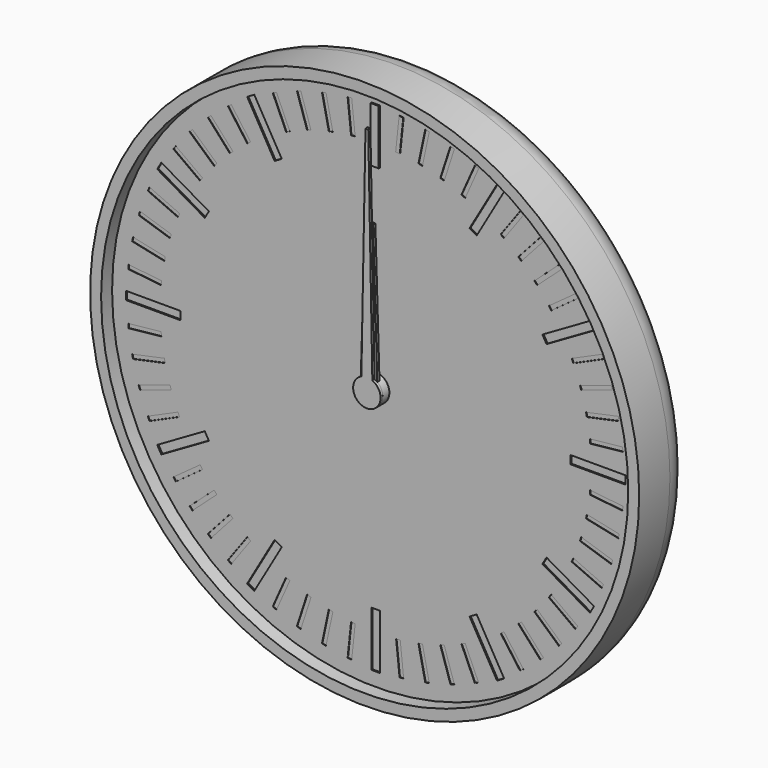
from build123d import *

# Parameters (mm, degrees)
F0_R      = 100
F1_DEPTH  = 24
F2_R      = 10
F3_T      = -4
F4_R      = 5
F4_R_2    = 3
F5_DEPTH  = 2
F6_DEPTH  = 19
F7_DEPTH  = 8
F9_DEPTH  = 4
F11_DEPTH = 4
F12_R     = 5
F12_R_2   = 3
F13_DEPTH = 2
F14_R     = 3
F15_DEPTH = 4
F17_DEPTH = 4
F18_R     = 3
F19_DEPTH = 2
F20_R     = 98
F20_R_2   = 5
F21_DEPTH = 1
F23_R     = 5
F23_R_2   = 3
F24_DEPTH = 2
F25_W     = 3
F25_H     = 20
F25_W_2   = 20
F25_H_2   = 3
F26_DEPTH = 0.5
F27_W     = 1.5
F27_H     = 12
F27_W_2   = 12
F27_H_2   = 1.5
F28_DEPTH = 0.2
F29_DEPTH = 1
F30_DEPTH = 0.4
F31_R     = 5
F31_R_2   = 3
F32_DEPTH = 5
F33_R     = 3
F34_DEPTH = 1
F36_DEPTH = 1


with BuildPart() as f1:
    # F0 (on Front) → F1 (new body)
    with BuildSketch(Plane.XZ):
        Circle(F0_R)
    extrude(amount=F1_DEPTH)

    # F2
    f2_edges = [f1.edges().sort_by_distance(p)[0] for p in [
        (-100, 0, 0),
    ]]
    fillet(f2_edges, radius=F2_R)

    # F3
    f3_openings = [f1.faces().sort_by_distance(p)[0] for p in [
        (0, -24, 0),
    ]]
    offset(amount=F3_T, openings=f3_openings)

    # F4 (on face) → F5 (join)
    with BuildSketch(Plane.XZ.offset(4)):
        Circle(F4_R)
        Circle(F4_R_2, mode=Mode.SUBTRACT)
        with Locations((40, 0)):
            Circle(F4_R)
        with Locations((40, 0)):
            Circle(F4_R_2, mode=Mode.SUBTRACT)
    extrude(amount=F5_DEPTH)


with BuildPart() as f6:
    # F6 (new): a face of the model
    f6_faces = [f1.part.faces().sort_by_distance(p)[0] for p in [
        (0, -4, 0),
    ]]
    extrude(f6_faces, amount=F6_DEPTH)

    # F8 (on face) → F9 (join)
    with BuildSketch(Plane.XZ.offset(6)):
        with BuildLine():
            ThreePointArc((9.2729637667, -1.3794085621), (9.3494561423, -0.6915886375), (9.375, 0))
            ThreePointArc((9.375, 0), (9.3494561423, 0.6915886375), (9.2729637667, 1.3794085621))
            ThreePointArc((9.2729637667, 1.3794085621), (8.9161548403, 2.8970343223), (8.3127812852, 4.3345463782))
            ThreePointArc((8.3127812852, 4.3345463782), (7.5845343223, 5.5104867402), (6.6911892658, 6.566476316))
            ThreePointArc((6.6911892658, 6.566476316), (5.5104867402, 7.5845343223), (4.1773988938, 8.3928519278))
            ThreePointArc((4.1773988938, 8.3928519278), (2.8970343223, 8.9161548403), (1.5536078905, 9.2453733036))
            ThreePointArc((1.5536078905, 9.2453733036), (0, 9.375), (-1.5536078905, 9.2453733036))
            ThreePointArc((-1.5536078905, 9.2453733036), (-2.8970343223, 8.9161548403), (-4.1773988938, 8.3928519278))
            ThreePointArc((-4.1773988938, 8.3928519278), (-5.5104867402, 7.5845343223), (-6.6911892658, 6.566476316))
            ThreePointArc((-6.6911892658, 6.566476316), (-7.5845343223, 5.5104867402), (-8.3127812852, 4.3345463782))
            ThreePointArc((-8.3127812852, 4.3345463782), (-8.9161548403, 2.8970343223), (-9.2729637667, 1.3794085621))
            ThreePointArc((-9.2729637667, 1.3794085621), (-9.375, 0), (-9.2729637667, -1.3794085621))
            ThreePointArc((-9.2729637667, -1.3794085621), (-8.9161548403, -2.8970343223), (-8.3127812852, -4.3345463782))
            ThreePointArc((-8.3127812852, -4.3345463782), (-7.5845343223, -5.5104867402), (-6.6911892658, -6.566476316))
            ThreePointArc((-6.6911892658, -6.566476316), (-5.5104867402, -7.5845343223), (-4.1773988938, -8.3928519278))
            ThreePointArc((-4.1773988938, -8.3928519278), (-2.8970343223, -8.9161548403), (-1.5536078905, -9.2453733036))
            ThreePointArc((-1.5536078905, -9.2453733036), (0, -9.375), (1.5536078905, -9.2453733036))
            ThreePointArc((1.5536078905, -9.2453733036), (2.8970343223, -8.9161548403), (4.1773988938, -8.3928519278))
            ThreePointArc((4.1773988938, -8.3928519278), (5.5104867402, -7.5845343223), (6.6911892658, -6.566476316))
            ThreePointArc((6.6911892658, -6.566476316), (7.5845343223, -5.5104867402), (8.3127812852, -4.3345463782))
            ThreePointArc((8.3127812852, -4.3345463782), (8.9161548403, -2.8970343223), (9.2729637667, -1.3794085621))
        make_face()
        with BuildLine():
            ThreePointArc((8.3127812852, 4.3345463782), (8.9161548403, 2.8970343223), (9.2729637667, 1.3794085621))
            Line((9.2729637667, 1.3794085621), (11.1823199426, 2.3946312492))
            Line((11.1823199426, 2.3946312492), (10.8182678729, 3.515068311))
            Line((10.8182678729, 3.515068311), (10.4542158031, 4.6355053728))
            Line((10.4542158031, 4.6355053728), (8.3127812852, 4.3345463782))
        make_face()
        with BuildLine():
            Line((11.1823199426, -2.3946312492), (9.2729637667, -1.3794085621))
            ThreePointArc((9.2729637667, -1.3794085621), (8.9161548403, -2.8970343223), (8.3127812852, -4.3345463782))
            Line((8.3127812852, -4.3345463782), (10.4542158031, -4.6355053728))
            Line((10.4542158031, -4.6355053728), (10.8182678729, -3.515068311))
            Line((10.8182678729, -3.515068311), (11.1823199426, -2.3946312492))
        make_face()
        with BuildLine():
            ThreePointArc((4.1773988938, 8.3928519278), (5.5104867402, 7.5845343223), (6.6911892658, 6.566476316))
            Line((6.6911892658, 6.566476316), (7.6391579371, 8.5101001246))
            Line((7.6391579371, 8.5101001246), (6.6860572448, 9.202568311))
            Line((6.6860572448, 9.202568311), (5.7329565525, 9.8950364974))
            Line((5.7329565525, 9.8950364974), (4.1773988938, 8.3928519278))
        make_face()
        with BuildLine():
            Line((7.6391579371, -8.5101001246), (6.6911892658, -6.566476316))
            ThreePointArc((6.6911892658, -6.566476316), (5.5104867402, -7.5845343223), (4.1773988938, -8.3928519278))
            Line((4.1773988938, -8.3928519278), (5.7329565525, -9.8950364974))
            Line((5.7329565525, -9.8950364974), (6.6860572448, -9.202568311))
            Line((6.6860572448, -9.202568311), (7.6391579371, -8.5101001246))
        make_face()
        with BuildLine():
            ThreePointArc((-1.5536078905, 9.2453733036), (0, 9.375), (1.5536078905, 9.2453733036))
            Line((1.5536078905, 9.2453733036), (1.1780972451, 11.375))
            Line((1.1780972451, 11.375), (0, 11.375))
            Line((0, 11.375), (-1.1780972451, 11.375))
            Line((-1.1780972451, 11.375), (-1.5536078905, 9.2453733036))
        make_face()
        with BuildLine():
            Line((1.1780972451, -11.375), (1.5536078905, -9.2453733036))
            ThreePointArc((1.5536078905, -9.2453733036), (0, -9.375), (-1.5536078905, -9.2453733036))
            Line((-1.5536078905, -9.2453733036), (-1.1780972451, -11.375))
            Line((-1.1780972451, -11.375), (0, -11.375))
            Line((0, -11.375), (1.1780972451, -11.375))
        make_face()
        with BuildLine():
            ThreePointArc((-6.6911892658, 6.566476316), (-5.5104867402, 7.5845343223), (-4.1773988938, 8.3928519278))
            Line((-4.1773988938, 8.3928519278), (-5.7329565525, 9.8950364974))
            Line((-5.7329565525, 9.8950364974), (-6.6860572448, 9.202568311))
            Line((-6.6860572448, 9.202568311), (-7.6391579371, 8.5101001246))
            Line((-7.6391579371, 8.5101001246), (-6.6911892658, 6.566476316))
        make_face()
        with BuildLine():
            Line((-5.7329565525, -9.8950364974), (-4.1773988938, -8.3928519278))
            ThreePointArc((-4.1773988938, -8.3928519278), (-5.5104867402, -7.5845343223), (-6.6911892658, -6.566476316))
            Line((-6.6911892658, -6.566476316), (-7.6391579371, -8.5101001246))
            Line((-7.6391579371, -8.5101001246), (-6.6860572448, -9.202568311))
            Line((-6.6860572448, -9.202568311), (-5.7329565525, -9.8950364974))
        make_face()
        with BuildLine():
            ThreePointArc((-9.2729637667, 1.3794085621), (-8.9161548403, 2.8970343223), (-8.3127812852, 4.3345463782))
            Line((-8.3127812852, 4.3345463782), (-10.4542158031, 4.6355053728))
            Line((-10.4542158031, 4.6355053728), (-10.8182678729, 3.515068311))
            Line((-10.8182678729, 3.515068311), (-11.1823199426, 2.3946312492))
            Line((-11.1823199426, 2.3946312492), (-9.2729637667, 1.3794085621))
        make_face()
        with BuildLine():
            Line((-10.4542158031, -4.6355053728), (-8.3127812852, -4.3345463782))
            ThreePointArc((-8.3127812852, -4.3345463782), (-8.9161548403, -2.8970343223), (-9.2729637667, -1.3794085621))
            Line((-9.2729637667, -1.3794085621), (-11.1823199426, -2.3946312492))
            Line((-11.1823199426, -2.3946312492), (-10.8182678729, -3.515068311))
            Line((-10.8182678729, -3.515068311), (-10.4542158031, -4.6355053728))
        make_face()
    extrude(amount=F9_DEPTH)

    # F35 (on face) → F36 (join)
    with BuildSketch(Plane.XZ.offset(23)):
        with BuildLine():
            ThreePointArc((-2, 4.582575695), (-2.7386127875, -4.1833001327), (5, 0))
            ThreePointArc((5, 0), (4.1833001327, 2.7386127875), (2, 4.582575695))
            ThreePointArc((2, 4.582575695), (0, 5), (-2, 4.582575695))
        make_face()
        with BuildLine():
            ThreePointArc((-2, 4.582575695), (0, 5), (2, 4.582575695))
            Line((2, 4.582575695), (0.5, 84.582575695))
            Line((0.5, 84.582575695), (0, 84.582575695))
            Line((0, 84.582575695), (-0.5, 84.582575695))
            Line((-0.5, 84.582575695), (-2, 4.582575695))
        make_face()
    extrude(amount=-F36_DEPTH)


with BuildPart() as f7:
    # F7 (new): a face of the model
    f7_faces = [f1.part.faces().sort_by_distance(p)[0] for p in [
        (40, -4, 0),
    ]]
    extrude(f7_faces, amount=F7_DEPTH)

    # F10 (on face) → F11 (join)
    with BuildSketch(Plane.XZ.offset(6)):
        with BuildLine():
            ThreePointArc((68.0829066802, -1.5381733945), (68.1144747006, -0.7693746225), (68.125, 0))
            ThreePointArc((68.125, 0), (68.1144747006, 0.7693746225), (68.0829066802, 1.5381733945))
            ThreePointArc((68.0829066802, 1.5381733945), (67.9709283072, 2.9398630294), (67.7890320221, 4.3342039956))
            ThreePointArc((67.7890320221, 4.3342039956), (67.5104012706, 5.8475163042), (67.1494235596, 7.3433252263))
            ThreePointArc((67.1494235596, 7.3433252263), (66.7484645208, 8.6911029668), (66.280643318, 10.0171558733))
            ThreePointArc((66.280643318, 10.0171558733), (65.6934659962, 11.4394680865), (65.0293803521, 12.8275385085))
            ThreePointArc((65.0293803521, 12.8275385085), (64.3569644814, 14.0625), (63.6236643925, 15.2623099717))
            ThreePointArc((63.6236643925, 15.2623099717), (62.7536029668, 16.5314602207), (61.815433119, 17.7511268046))
            ThreePointArc((61.815433119, 17.7511268046), (60.9009482166, 18.8192983038), (59.934217974, 19.8404278876))
            ThreePointArc((59.934217974, 19.8404278876), (58.8192983038, 20.9009482166), (57.6480467764, 21.8989056799))
            ThreePointArc((57.6480467764, 21.8989056799), (56.5314602207, 22.7536029668), (55.3735505752, 23.5514238999))
            ThreePointArc((55.3735505752, 23.5514238999), (54.0625, 24.3569644814), (52.709356105, 25.0895972944))
            ThreePointArc((52.709356105, 25.0895972944), (51.4394680865, 25.6934659962), (50.1409852457, 26.2331096755))
            ThreePointArc((50.1409852457, 26.2331096755), (48.6911029668, 26.7484645208), (47.2152055856, 27.1837531139))
            ThreePointArc((47.2152055856, 27.1837531139), (45.8475163042, 27.5104012706), (44.4652101991, 27.7682826779))
            ThreePointArc((44.4652101991, 27.7682826779), (42.9398630294, 27.9709283072), (41.4057159597, 28.0898484802))
            ThreePointArc((41.4057159597, 28.0898484802), (40, 28.125), (38.5942840403, 28.0898484802))
            ThreePointArc((38.5942840403, 28.0898484802), (37.0601369706, 27.9709283072), (35.5347898009, 27.7682826779))
            ThreePointArc((35.5347898009, 27.7682826779), (34.1524836958, 27.5104012706), (32.7847944144, 27.1837531139))
            ThreePointArc((32.7847944144, 27.1837531139), (31.3088970332, 26.7484645208), (29.8590147543, 26.2331096755))
            ThreePointArc((29.8590147543, 26.2331096755), (28.5605319135, 25.6934659962), (27.290643895, 25.0895972944))
            ThreePointArc((27.290643895, 25.0895972944), (25.9375, 24.3569644814), (24.6264494248, 23.5514238999))
            ThreePointArc((24.6264494248, 23.5514238999), (23.4685397793, 22.7536029668), (22.3519532236, 21.8989056799))
            ThreePointArc((22.3519532236, 21.8989056799), (21.1807016962, 20.9009482166), (20.065782026, 19.8404278876))
            ThreePointArc((20.065782026, 19.8404278876), (19.0990517834, 18.8192983038), (18.184566881, 17.7511268046))
            ThreePointArc((18.184566881, 17.7511268046), (17.2463970332, 16.5314602207), (16.3763356075, 15.2623099717))
            ThreePointArc((16.3763356075, 15.2623099717), (15.6430355186, 14.0625), (14.9706196479, 12.8275385085))
            ThreePointArc((14.9706196479, 12.8275385085), (14.3065340038, 11.4394680865), (13.719356682, 10.0171558733))
            ThreePointArc((13.719356682, 10.0171558733), (13.2515354792, 8.6911029668), (12.8505764404, 7.3433252263))
            ThreePointArc((12.8505764404, 7.3433252263), (12.4895987294, 5.8475163042), (12.2109679779, 4.3342039956))
            ThreePointArc((12.2109679779, 4.3342039956), (12.0290716928, 2.9398630294), (11.9170933198, 1.5381733945))
            ThreePointArc((11.9170933198, 1.5381733945), (11.875, 0), (11.9170933198, -1.5381733945))
            ThreePointArc((11.9170933198, -1.5381733945), (12.0290716928, -2.9398630294), (12.2109679779, -4.3342039956))
            ThreePointArc((12.2109679779, -4.3342039956), (12.4895987294, -5.8475163042), (12.8505764404, -7.3433252263))
            ThreePointArc((12.8505764404, -7.3433252263), (13.2515354792, -8.6911029668), (13.719356682, -10.0171558733))
            ThreePointArc((13.719356682, -10.0171558733), (14.3065340038, -11.4394680865), (14.9706196479, -12.8275385085))
            ThreePointArc((14.9706196479, -12.8275385085), (15.6430355186, -14.0625), (16.3763356075, -15.2623099717))
            ThreePointArc((16.3763356075, -15.2623099717), (17.2463970332, -16.5314602207), (18.184566881, -17.7511268046))
            ThreePointArc((18.184566881, -17.7511268046), (19.0990517834, -18.8192983038), (20.065782026, -19.8404278876))
            ThreePointArc((20.065782026, -19.8404278876), (21.1807016962, -20.9009482166), (22.3519532236, -21.8989056799))
            ThreePointArc((22.3519532236, -21.8989056799), (23.4685397793, -22.7536029668), (24.6264494248, -23.5514238999))
            ThreePointArc((24.6264494248, -23.5514238999), (25.9375, -24.3569644814), (27.290643895, -25.0895972944))
            ThreePointArc((27.290643895, -25.0895972944), (28.5605319135, -25.6934659962), (29.8590147543, -26.2331096755))
            ThreePointArc((29.8590147543, -26.2331096755), (31.3088970332, -26.7484645208), (32.7847944144, -27.1837531139))
            ThreePointArc((32.7847944144, -27.1837531139), (34.1524836958, -27.5104012706), (35.5347898009, -27.7682826779))
            ThreePointArc((35.5347898009, -27.7682826779), (37.0601369706, -27.9709283072), (38.5942840403, -28.0898484802))
            ThreePointArc((38.5942840403, -28.0898484802), (40, -28.125), (41.4057159597, -28.0898484802))
            ThreePointArc((41.4057159597, -28.0898484802), (42.9398630294, -27.9709283072), (44.4652101991, -27.7682826779))
            ThreePointArc((44.4652101991, -27.7682826779), (45.8475163042, -27.5104012706), (47.2152055856, -27.1837531139))
            ThreePointArc((47.2152055856, -27.1837531139), (48.6911029668, -26.7484645208), (50.1409852457, -26.2331096755))
            ThreePointArc((50.1409852457, -26.2331096755), (51.4394680865, -25.6934659962), (52.709356105, -25.0895972944))
            ThreePointArc((52.709356105, -25.0895972944), (54.0625, -24.3569644814), (55.3735505752, -23.5514238999))
            ThreePointArc((55.3735505752, -23.5514238999), (56.5314602207, -22.7536029668), (57.6480467764, -21.8989056799))
            ThreePointArc((57.6480467764, -21.8989056799), (58.8192983038, -20.9009482166), (59.934217974, -19.8404278876))
            ThreePointArc((59.934217974, -19.8404278876), (60.9009482166, -18.8192983038), (61.815433119, -17.7511268046))
            ThreePointArc((61.815433119, -17.7511268046), (62.7536029668, -16.5314602207), (63.6236643925, -15.2623099717))
            ThreePointArc((63.6236643925, -15.2623099717), (64.3569644814, -14.0625), (65.0293803521, -12.8275385085))
            ThreePointArc((65.0293803521, -12.8275385085), (65.6934659962, -11.4394680865), (66.280643318, -10.0171558733))
            ThreePointArc((66.280643318, -10.0171558733), (66.7484645208, -8.6911029668), (67.1494235596, -7.3433252263))
            ThreePointArc((67.1494235596, -7.3433252263), (67.5104012706, -5.8475163042), (67.7890320221, -4.3342039956))
            ThreePointArc((67.7890320221, -4.3342039956), (67.9709283072, -2.9398630294), (68.0829066802, -1.5381733945))
        make_face()
        with BuildLine():
            ThreePointArc((68.0829066802, 1.5381733945), (68.1144747006, 0.7693746225), (68.125, 0))
            ThreePointArc((68.125, 0), (68.1144747006, -0.7693746225), (68.0829066802, -1.5381733945))
            Line((68.0829066802, -1.5381733945), (70.125, -1.1780972451))
            Line((70.125, -1.1780972451), (70.125, 0))
            Line((70.125, 0), (70.125, 1.1780972451))
            Line((70.125, 1.1780972451), (68.0829066802, 1.5381733945))
        make_face()
        with BuildLine():
            ThreePointArc((67.1494235596, 7.3433252263), (67.5104012706, 5.8475163042), (67.7890320221, 4.3342039956))
            Line((67.7890320221, 4.3342039956), (69.7116366623, 5.1109866922))
            Line((69.7116366623, 5.1109866922), (69.4666964721, 6.2633396859))
            Line((69.4666964721, 6.2633396859), (69.2217562819, 7.4156926796))
            Line((69.2217562819, 7.4156926796), (67.1494235596, 7.3433252263))
        make_face()
        with BuildLine():
            Line((69.7116366623, -5.1109866922), (67.7890320221, -4.3342039956))
            ThreePointArc((67.7890320221, -4.3342039956), (67.5104012706, -5.8475163042), (67.1494235596, -7.3433252263))
            Line((67.1494235596, -7.3433252263), (69.2217562819, -7.4156926796))
            Line((69.2217562819, -7.4156926796), (69.4666964721, -6.2633396859))
            Line((69.4666964721, -6.2633396859), (69.7116366623, -5.1109866922))
        make_face()
        with BuildLine():
            ThreePointArc((65.0293803521, 12.8275385085), (65.6934659962, 11.4394680865), (66.280643318, 10.0171558733))
            Line((66.280643318, 10.0171558733), (67.9997322302, 11.1766959857))
            Line((67.9997322302, 11.1766959857), (67.5205569115, 12.2529413727))
            Line((67.5205569115, 12.2529413727), (67.0413815928, 13.3291867596))
            Line((67.0413815928, 13.3291867596), (65.0293803521, 12.8275385085))
        make_face()
        with BuildLine():
            Line((67.9997322302, -11.1766959857), (66.280643318, -10.0171558733))
            ThreePointArc((66.280643318, -10.0171558733), (65.6934659962, -11.4394680865), (65.0293803521, -12.8275385085))
            Line((65.0293803521, -12.8275385085), (67.0413815928, -13.3291867596))
            Line((67.0413815928, -13.3291867596), (67.5205569115, -12.2529413727))
            Line((67.5205569115, -12.2529413727), (67.9997322302, -11.1766959857))
        make_face()
        with BuildLine():
            ThreePointArc((61.815433119, 17.7511268046), (62.7536029668, 16.5314602207), (63.6236643925, 15.2623099717))
            Line((63.6236643925, 15.2623099717), (65.064105142, 16.753930033))
            Line((65.064105142, 16.753930033), (64.3716369555, 17.7070307253))
            Line((64.3716369555, 17.7070307253), (63.6791687691, 18.6601314176))
            Line((63.6791687691, 18.6601314176), (61.815433119, 17.7511268046))
        make_face()
        with BuildLine():
            Line((65.064105142, -16.753930033), (63.6236643925, -15.2623099717))
            ThreePointArc((63.6236643925, -15.2623099717), (62.7536029668, -16.5314602207), (61.815433119, -17.7511268046))
            Line((61.815433119, -17.7511268046), (63.6791687691, -18.6601314176))
            Line((63.6791687691, -18.6601314176), (64.3716369555, -17.7070307253))
            Line((64.3716369555, -17.7070307253), (65.064105142, -16.753930033))
        make_face()
        with BuildLine():
            ThreePointArc((57.6480467764, 21.8989056799), (58.8192983038, 20.9009482166), (59.934217974, 19.8404278876))
            Line((59.934217974, 19.8404278876), (61.0330563882, 21.5989369435))
            Line((61.0330563882, 21.5989369435), (60.1575595166, 22.3872378675))
            Line((60.1575595166, 22.3872378675), (59.282062645, 23.1755387915))
            Line((59.282062645, 23.1755387915), (57.6480467764, 21.8989056799))
        make_face()
        with BuildLine():
            Line((61.0330563882, -21.5989369435), (59.934217974, -19.8404278876))
            ThreePointArc((59.934217974, -19.8404278876), (58.8192983038, -20.9009482166), (57.6480467764, -21.8989056799))
            Line((57.6480467764, -21.8989056799), (59.282062645, -23.1755387915))
            Line((59.282062645, -23.1755387915), (60.1575595166, -22.3872378675))
            Line((60.1575595166, -22.3872378675), (61.0330563882, -21.5989369435))
        make_face()
        with BuildLine():
            ThreePointArc((52.709356105, 25.0895972944), (54.0625, 24.3569644814), (55.3735505752, 23.5514238999))
            Line((55.3735505752, 23.5514238999), (56.0827621424, 25.4999666665))
            Line((56.0827621424, 25.4999666665), (55.0625, 26.089015289))
            Line((55.0625, 26.089015289), (54.0422378576, 26.6780639116))
            Line((54.0422378576, 26.6780639116), (52.709356105, 25.0895972944))
        make_face()
        with BuildLine():
            Line((56.0827621424, -25.4999666665), (55.3735505752, -23.5514238999))
            ThreePointArc((55.3735505752, -23.5514238999), (54.0625, -24.3569644814), (52.709356105, -25.0895972944))
            Line((52.709356105, -25.0895972944), (54.0422378576, -26.6780639116))
            Line((54.0422378576, -26.6780639116), (55.0625, -26.089015289))
            Line((55.0625, -26.089015289), (56.0827621424, -25.4999666665))
        make_face()
        with BuildLine():
            ThreePointArc((47.2152055856, 27.1837531139), (48.6911029668, 26.7484645208), (50.1409852457, 26.2331096755))
            Line((50.1409852457, 26.2331096755), (50.4295740173, 28.2865254836))
            Line((50.4295740173, 28.2865254836), (49.3091369555, 28.6505775534))
            Line((49.3091369555, 28.6505775534), (48.1886998938, 29.0146296232))
            Line((48.1886998938, 29.0146296232), (47.2152055856, 27.1837531139))
        make_face()
        with BuildLine():
            Line((50.4295740173, -28.2865254836), (50.1409852457, -26.2331096755))
            ThreePointArc((50.1409852457, -26.2331096755), (48.6911029668, -26.7484645208), (47.2152055856, -27.1837531139))
            Line((47.2152055856, -27.1837531139), (48.1886998938, -29.0146296232))
            Line((48.1886998938, -29.0146296232), (49.3091369555, -28.6505775534))
            Line((49.3091369555, -28.6505775534), (50.4295740173, -28.2865254836))
        make_face()
        with BuildLine():
            ThreePointArc((41.4057159597, 28.0898484802), (42.9398630294, 27.9709283072), (44.4652101991, 27.7682826779))
            Line((44.4652101991, 27.7682826779), (44.3205634611, 29.8368274034))
            Line((44.3205634611, 29.8368274034), (43.1489199559, 29.959972098))
            Line((43.1489199559, 29.959972098), (41.9772764508, 30.0831167926))
            Line((41.9772764508, 30.0831167926), (41.4057159597, 28.0898484802))
        make_face()
        with BuildLine():
            Line((44.3205634611, -29.8368274034), (44.4652101991, -27.7682826779))
            ThreePointArc((44.4652101991, -27.7682826779), (42.9398630294, -27.9709283072), (41.4057159597, -28.0898484802))
            Line((41.4057159597, -28.0898484802), (41.9772764508, -30.0831167926))
            Line((41.9772764508, -30.0831167926), (43.1489199559, -29.959972098))
            Line((43.1489199559, -29.959972098), (44.3205634611, -29.8368274034))
        make_face()
        with BuildLine():
            ThreePointArc((35.5347898009, 27.7682826779), (37.0601369706, 27.9709283072), (38.5942840403, 28.0898484802))
            Line((38.5942840403, 28.0898484802), (38.0227235492, 30.0831167926))
            Line((38.0227235492, 30.0831167926), (36.8510800441, 29.959972098))
            Line((36.8510800441, 29.959972098), (35.6794365389, 29.8368274034))
            Line((35.6794365389, 29.8368274034), (35.5347898009, 27.7682826779))
        make_face()
        with BuildLine():
            Line((38.0227235492, -30.0831167926), (38.5942840403, -28.0898484802))
            ThreePointArc((38.5942840403, -28.0898484802), (37.0601369706, -27.9709283072), (35.5347898009, -27.7682826779))
            Line((35.5347898009, -27.7682826779), (35.6794365389, -29.8368274034))
            Line((35.6794365389, -29.8368274034), (36.8510800441, -29.959972098))
            Line((36.8510800441, -29.959972098), (38.0227235492, -30.0831167926))
        make_face()
        with BuildLine():
            ThreePointArc((29.8590147543, 26.2331096755), (31.3088970332, 26.7484645208), (32.7847944144, 27.1837531139))
            Line((32.7847944144, 27.1837531139), (31.8113001062, 29.0146296232))
            Line((31.8113001062, 29.0146296232), (30.6908630445, 28.6505775534))
            Line((30.6908630445, 28.6505775534), (29.5704259827, 28.2865254836))
            Line((29.5704259827, 28.2865254836), (29.8590147543, 26.2331096755))
        make_face()
        with BuildLine():
            Line((31.8113001062, -29.0146296232), (32.7847944144, -27.1837531139))
            ThreePointArc((32.7847944144, -27.1837531139), (31.3088970332, -26.7484645208), (29.8590147543, -26.2331096755))
            Line((29.8590147543, -26.2331096755), (29.5704259827, -28.2865254836))
            Line((29.5704259827, -28.2865254836), (30.6908630445, -28.6505775534))
            Line((30.6908630445, -28.6505775534), (31.8113001062, -29.0146296232))
        make_face()
        with BuildLine():
            ThreePointArc((24.6264494248, 23.5514238999), (25.9375, 24.3569644814), (27.290643895, 25.0895972944))
            Line((27.290643895, 25.0895972944), (25.9577621424, 26.6780639116))
            Line((25.9577621424, 26.6780639116), (24.9375, 26.089015289))
            Line((24.9375, 26.089015289), (23.9172378576, 25.4999666665))
            Line((23.9172378576, 25.4999666665), (24.6264494248, 23.5514238999))
        make_face()
        with BuildLine():
            Line((25.9577621424, -26.6780639116), (27.290643895, -25.0895972944))
            ThreePointArc((27.290643895, -25.0895972944), (25.9375, -24.3569644814), (24.6264494248, -23.5514238999))
            Line((24.6264494248, -23.5514238999), (23.9172378576, -25.4999666665))
            Line((23.9172378576, -25.4999666665), (24.9375, -26.089015289))
            Line((24.9375, -26.089015289), (25.9577621424, -26.6780639116))
        make_face()
        with BuildLine():
            ThreePointArc((20.065782026, 19.8404278876), (21.1807016962, 20.9009482166), (22.3519532236, 21.8989056799))
            Line((22.3519532236, 21.8989056799), (20.717937355, 23.1755387915))
            Line((20.717937355, 23.1755387915), (19.8424404834, 22.3872378675))
            Line((19.8424404834, 22.3872378675), (18.9669436118, 21.5989369435))
            Line((18.9669436118, 21.5989369435), (20.065782026, 19.8404278876))
        make_face()
        with BuildLine():
            Line((20.717937355, -23.1755387915), (22.3519532236, -21.8989056799))
            ThreePointArc((22.3519532236, -21.8989056799), (21.1807016962, -20.9009482166), (20.065782026, -19.8404278876))
            Line((20.065782026, -19.8404278876), (18.9669436118, -21.5989369435))
            Line((18.9669436118, -21.5989369435), (19.8424404834, -22.3872378675))
            Line((19.8424404834, -22.3872378675), (20.717937355, -23.1755387915))
        make_face()
        with BuildLine():
            ThreePointArc((16.3763356075, 15.2623099717), (17.2463970332, 16.5314602207), (18.184566881, 17.7511268046))
            Line((18.184566881, 17.7511268046), (16.3208312309, 18.6601314176))
            Line((16.3208312309, 18.6601314176), (15.6283630445, 17.7070307253))
            Line((15.6283630445, 17.7070307253), (14.935894858, 16.753930033))
            Line((14.935894858, 16.753930033), (16.3763356075, 15.2623099717))
        make_face()
        with BuildLine():
            Line((16.3208312309, -18.6601314176), (18.184566881, -17.7511268046))
            ThreePointArc((18.184566881, -17.7511268046), (17.2463970332, -16.5314602207), (16.3763356075, -15.2623099717))
            Line((16.3763356075, -15.2623099717), (14.935894858, -16.753930033))
            Line((14.935894858, -16.753930033), (15.6283630445, -17.7070307253))
            Line((15.6283630445, -17.7070307253), (16.3208312309, -18.6601314176))
        make_face()
        with BuildLine():
            ThreePointArc((13.719356682, 10.0171558733), (14.3065340038, 11.4394680865), (14.9706196479, 12.8275385085))
            Line((14.9706196479, 12.8275385085), (12.9586184072, 13.3291867596))
            Line((12.9586184072, 13.3291867596), (12.4794430885, 12.2529413727))
            Line((12.4794430885, 12.2529413727), (12.0002677698, 11.1766959857))
            Line((12.0002677698, 11.1766959857), (13.719356682, 10.0171558733))
        make_face()
        with BuildLine():
            Line((12.9586184072, -13.3291867596), (14.9706196479, -12.8275385085))
            ThreePointArc((14.9706196479, -12.8275385085), (14.3065340038, -11.4394680865), (13.719356682, -10.0171558733))
            Line((13.719356682, -10.0171558733), (12.0002677698, -11.1766959857))
            Line((12.0002677698, -11.1766959857), (12.4794430885, -12.2529413727))
            Line((12.4794430885, -12.2529413727), (12.9586184072, -13.3291867596))
        make_face()
        with BuildLine():
            ThreePointArc((12.2109679779, 4.3342039956), (12.4895987294, 5.8475163042), (12.8505764404, 7.3433252263))
            Line((12.8505764404, 7.3433252263), (10.7782437181, 7.4156926796))
            Line((10.7782437181, 7.4156926796), (10.5333035279, 6.2633396859))
            Line((10.5333035279, 6.2633396859), (10.2883633377, 5.1109866922))
            Line((10.2883633377, 5.1109866922), (12.2109679779, 4.3342039956))
        make_face()
        with BuildLine():
            Line((10.7782437181, -7.4156926796), (12.8505764404, -7.3433252263))
            ThreePointArc((12.8505764404, -7.3433252263), (12.4895987294, -5.8475163042), (12.2109679779, -4.3342039956))
            Line((12.2109679779, -4.3342039956), (10.2883633377, -5.1109866922))
            Line((10.2883633377, -5.1109866922), (10.5333035279, -6.2633396859))
            Line((10.5333035279, -6.2633396859), (10.7782437181, -7.4156926796))
        make_face()
        with BuildLine():
            ThreePointArc((11.9170933198, -1.5381733945), (11.875, 0), (11.9170933198, 1.5381733945))
            Line((11.9170933198, 1.5381733945), (9.875, 1.1780972451))
            Line((9.875, 1.1780972451), (9.875, 0))
            Line((9.875, 0), (9.875, -1.1780972451))
            Line((9.875, -1.1780972451), (11.9170933198, -1.5381733945))
        make_face()
    extrude(amount=F11_DEPTH)

    # F16 (on face) → F17 (join)
    with BuildSketch(Plane.XZ.offset(12)):
        with BuildLine():
            ThreePointArc((47.4288750323, -1.0304444454), (47.4821976298, -0.5164480894), (47.5, 0))
            ThreePointArc((47.5, 0), (47.4821976298, 0.5164480894), (47.4288750323, 1.0304444454))
            ThreePointArc((47.4288750323, 1.0304444454), (47.1329238722, 2.3176274578), (46.6157661985, 3.532936117))
            ThreePointArc((46.6157661985, 3.532936117), (46.0676274578, 4.4083893922), (45.4044061018, 5.2002302532))
            ThreePointArc((45.4044061018, 5.2002302532), (44.4083893922, 6.0676274578), (43.2756595386, 6.7468551628))
            ThreePointArc((43.2756595386, 6.7468551628), (42.3176274578, 7.1329238722), (41.3156377295, 7.3837048536))
            ThreePointArc((41.3156377295, 7.3837048536), (40, 7.5), (38.6843622705, 7.3837048536))
            ThreePointArc((38.6843622705, 7.3837048536), (37.6823725422, 7.1329238722), (36.7243404614, 6.7468551628))
            ThreePointArc((36.7243404614, 6.7468551628), (35.5916106078, 6.0676274578), (34.5955938982, 5.2002302532))
            ThreePointArc((34.5955938982, 5.2002302532), (33.9323725422, 4.4083893922), (33.3842338015, 3.532936117))
            ThreePointArc((33.3842338015, 3.532936117), (32.8670761278, 2.3176274578), (32.5711249677, 1.0304444454))
            ThreePointArc((32.5711249677, 1.0304444454), (32.5, 0), (32.5711249677, -1.0304444454))
            ThreePointArc((32.5711249677, -1.0304444454), (32.8670761278, -2.3176274578), (33.3842338015, -3.532936117))
            ThreePointArc((33.3842338015, -3.532936117), (33.9323725422, -4.4083893922), (34.5955938982, -5.2002302532))
            ThreePointArc((34.5955938982, -5.2002302532), (35.5916106078, -6.0676274578), (36.7243404614, -6.7468551628))
            ThreePointArc((36.7243404614, -6.7468551628), (37.6823725422, -7.1329238722), (38.6843622705, -7.3837048536))
            ThreePointArc((38.6843622705, -7.3837048536), (40, -7.5), (41.3156377295, -7.3837048536))
            ThreePointArc((41.3156377295, -7.3837048536), (42.3176274578, -7.1329238722), (43.2756595386, -6.7468551628))
            ThreePointArc((43.2756595386, -6.7468551628), (44.4083893922, -6.0676274578), (45.4044061018, -5.2002302532))
            ThreePointArc((45.4044061018, -5.2002302532), (46.0676274578, -4.4083893922), (46.6157661985, -3.532936117))
            ThreePointArc((46.6157661985, -3.532936117), (47.1329238722, -2.3176274578), (47.4288750323, -1.0304444454))
        make_face()
        with BuildLine():
            ThreePointArc((46.6157661985, 3.532936117), (47.1329238722, 2.3176274578), (47.4288750323, 1.0304444454))
            Line((47.4288750323, 1.0304444454), (49.3262785606, 2.0393117971))
            Line((49.3262785606, 2.0393117971), (48.743795249, 3.832011096))
            Line((48.743795249, 3.832011096), (46.6157661985, 3.532936117))
        make_face()
        with BuildLine():
            Line((49.3262785606, -2.0393117971), (47.4288750323, -1.0304444454))
            ThreePointArc((47.4288750323, -1.0304444454), (47.1329238722, -2.3176274578), (46.6157661985, -3.532936117))
            Line((46.6157661985, -3.532936117), (48.743795249, -3.832011096))
            Line((48.743795249, -3.832011096), (49.3262785606, -2.0393117971))
        make_face()
        with BuildLine():
            ThreePointArc((43.2756595386, 6.7468551628), (44.4083893922, 6.0676274578), (45.4044061018, 5.2002302532))
            Line((45.4044061018, 5.2002302532), (46.3464404506, 7.1316868974))
            Line((46.3464404506, 7.1316868974), (44.8214793429, 8.2396359957))
            Line((44.8214793429, 8.2396359957), (43.2756595386, 6.7468551628))
        make_face()
        with BuildLine():
            Line((46.3464404506, -7.1316868974), (45.4044061018, -5.2002302532))
            ThreePointArc((45.4044061018, -5.2002302532), (44.4083893922, -6.0676274578), (43.2756595386, -6.7468551628))
            Line((43.2756595386, -6.7468551628), (44.8214793429, -8.2396359957))
            Line((44.8214793429, -8.2396359957), (46.3464404506, -7.1316868974))
        make_face()
        with BuildLine():
            ThreePointArc((38.6843622705, 7.3837048536), (40, 7.5), (41.3156377295, 7.3837048536))
            Line((41.3156377295, 7.3837048536), (40.9424777961, 9.5))
            Line((40.9424777961, 9.5), (39.0575222039, 9.5))
            Line((39.0575222039, 9.5), (38.6843622705, 7.3837048536))
        make_face()
        with BuildLine():
            Line((40.9424777961, -9.5), (41.3156377295, -7.3837048536))
            ThreePointArc((41.3156377295, -7.3837048536), (40, -7.5), (38.6843622705, -7.3837048536))
            Line((38.6843622705, -7.3837048536), (39.0575222039, -9.5))
            Line((39.0575222039, -9.5), (40.9424777961, -9.5))
        make_face()
        with BuildLine():
            ThreePointArc((34.5955938982, 5.2002302532), (35.5916106078, 6.0676274578), (36.7243404614, 6.7468551628))
            Line((36.7243404614, 6.7468551628), (35.1785206571, 8.2396359957))
            Line((35.1785206571, 8.2396359957), (33.6535595494, 7.1316868974))
            Line((33.6535595494, 7.1316868974), (34.5955938982, 5.2002302532))
        make_face()
        with BuildLine():
            Line((35.1785206571, -8.2396359957), (36.7243404614, -6.7468551628))
            ThreePointArc((36.7243404614, -6.7468551628), (35.5916106078, -6.0676274578), (34.5955938982, -5.2002302532))
            Line((34.5955938982, -5.2002302532), (33.6535595494, -7.1316868974))
            Line((33.6535595494, -7.1316868974), (35.1785206571, -8.2396359957))
        make_face()
        with BuildLine():
            ThreePointArc((32.5711249677, 1.0304444454), (32.8670761278, 2.3176274578), (33.3842338015, 3.532936117))
            Line((33.3842338015, 3.532936117), (31.256204751, 3.832011096))
            Line((31.256204751, 3.832011096), (30.6737214394, 2.0393117971))
            Line((30.6737214394, 2.0393117971), (32.5711249677, 1.0304444454))
        make_face()
        with BuildLine():
            Line((31.256204751, -3.832011096), (33.3842338015, -3.532936117))
            ThreePointArc((33.3842338015, -3.532936117), (32.8670761278, -2.3176274578), (32.5711249677, -1.0304444454))
            Line((32.5711249677, -1.0304444454), (30.6737214394, -2.0393117971))
            Line((30.6737214394, -2.0393117971), (31.256204751, -3.832011096))
        make_face()
    extrude(amount=F17_DEPTH)

    # F18 (on face) → F19 (join)
    with BuildSketch(Plane.XZ.offset(16)):
        with Locations((40, 0)):
            Circle(F18_R)
    extrude(amount=F19_DEPTH)


with BuildPart() as f13:
    # F12 (on face) → F13 (new body)
    with BuildSketch(Plane.XZ.offset(10)):
        Circle(F12_R)
        Circle(F12_R_2, mode=Mode.SUBTRACT)
    extrude(amount=F13_DEPTH)

    # F14 (on face) → F15 (join)
    with BuildSketch(Plane.XZ.offset(12)):
        with BuildLine():
            ThreePointArc((29.9718156995, -1.3001014101), (29.9929530972, -0.6502034357), (30, 0))
            ThreePointArc((30, 0), (29.9929530972, 0.6502034357), (29.9718156995, 1.3001014101))
            ThreePointArc((29.9718156995, 1.3001014101), (29.907520012, 2.3537728718), (29.8061935814, 3.4045299509))
            ThreePointArc((29.8061935814, 3.4045299509), (29.6306502179, 4.6930339512), (29.3994322443, 5.9727199596))
            ThreePointArc((29.3994322443, 5.9727199596), (29.1710976119, 7.0033609157), (28.9066440563, 8.0253304855))
            ThreePointArc((28.9066440563, 8.0253304855), (28.5316954889, 9.2705098312), (28.1031371961, 10.4982703213))
            ThreePointArc((28.1031371961, 10.4982703213), (27.7163859753, 11.480502971), (27.2953170189, 12.448520749))
            ThreePointArc((27.2953170189, 12.448520749), (26.7301957257, 13.6197149922), (26.1148496411, 14.765318426))
            ThreePointArc((26.1148496411, 14.765318426), (25.5792049306, 15.6749569415), (25.0118886885, 16.5651871174))
            ThreePointArc((25.0118886885, 16.5651871174), (24.2705098312, 17.6335575688), (23.4835278178, 18.6687953878))
            ThreePointArc((23.4835278178, 18.6687953878), (22.812178968, 19.4834414499), (22.1125846489, 20.2739636023))
            ThreePointArc((22.1125846489, 20.2739636023), (21.2132034356, 21.2132034356), (20.2739636023, 22.1125846489))
            ThreePointArc((20.2739636023, 22.1125846489), (19.4834414499, 22.812178968), (18.6687953878, 23.4835278178))
            ThreePointArc((18.6687953878, 23.4835278178), (17.6335575688, 24.2705098312), (16.5651871174, 25.0118886885))
            ThreePointArc((16.5651871174, 25.0118886885), (15.6749569415, 25.5792049306), (14.765318426, 26.1148496411))
            ThreePointArc((14.765318426, 26.1148496411), (13.6197149922, 26.7301957257), (12.448520749, 27.2953170189))
            ThreePointArc((12.448520749, 27.2953170189), (11.480502971, 27.7163859753), (10.4982703213, 28.1031371961))
            ThreePointArc((10.4982703213, 28.1031371961), (9.2705098312, 28.5316954889), (8.0253304855, 28.9066440563))
            ThreePointArc((8.0253304855, 28.9066440563), (7.0033609157, 29.1710976119), (5.9727199596, 29.3994322443))
            ThreePointArc((5.9727199596, 29.3994322443), (4.6930339512, 29.6306502179), (3.4045299509, 29.8061935814))
            ThreePointArc((3.4045299509, 29.8061935814), (2.3537728718, 29.907520012), (1.3001014101, 29.9718156995))
            ThreePointArc((1.3001014101, 29.9718156995), (0, 30), (-1.3001014101, 29.9718156995))
            ThreePointArc((-1.3001014101, 29.9718156995), (-2.3537728718, 29.907520012), (-3.4045299509, 29.8061935814))
            ThreePointArc((-3.4045299509, 29.8061935814), (-4.6930339512, 29.6306502179), (-5.9727199596, 29.3994322443))
            ThreePointArc((-5.9727199596, 29.3994322443), (-7.0033609157, 29.1710976119), (-8.0253304855, 28.9066440563))
            ThreePointArc((-8.0253304855, 28.9066440563), (-9.2705098312, 28.5316954889), (-10.4982703213, 28.1031371961))
            ThreePointArc((-10.4982703213, 28.1031371961), (-11.480502971, 27.7163859753), (-12.448520749, 27.2953170189))
            ThreePointArc((-12.448520749, 27.2953170189), (-13.6197149922, 26.7301957257), (-14.765318426, 26.1148496411))
            ThreePointArc((-14.765318426, 26.1148496411), (-15.6749569415, 25.5792049306), (-16.5651871174, 25.0118886885))
            ThreePointArc((-16.5651871174, 25.0118886885), (-17.6335575688, 24.2705098312), (-18.6687953878, 23.4835278178))
            ThreePointArc((-18.6687953878, 23.4835278178), (-19.4834414499, 22.812178968), (-20.2739636023, 22.1125846489))
            ThreePointArc((-20.2739636023, 22.1125846489), (-21.2132034356, 21.2132034356), (-22.1125846489, 20.2739636023))
            ThreePointArc((-22.1125846489, 20.2739636023), (-22.812178968, 19.4834414499), (-23.4835278178, 18.6687953878))
            ThreePointArc((-23.4835278178, 18.6687953878), (-24.2705098312, 17.6335575688), (-25.0118886885, 16.5651871174))
            ThreePointArc((-25.0118886885, 16.5651871174), (-25.5792049306, 15.6749569415), (-26.1148496411, 14.765318426))
            ThreePointArc((-26.1148496411, 14.765318426), (-26.7301957257, 13.6197149922), (-27.2953170189, 12.448520749))
            ThreePointArc((-27.2953170189, 12.448520749), (-27.7163859753, 11.480502971), (-28.1031371961, 10.4982703213))
            ThreePointArc((-28.1031371961, 10.4982703213), (-28.5316954889, 9.2705098312), (-28.9066440563, 8.0253304855))
            ThreePointArc((-28.9066440563, 8.0253304855), (-29.1710976119, 7.0033609157), (-29.3994322443, 5.9727199596))
            ThreePointArc((-29.3994322443, 5.9727199596), (-29.6306502179, 4.6930339512), (-29.8061935814, 3.4045299509))
            ThreePointArc((-29.8061935814, 3.4045299509), (-29.907520012, 2.3537728718), (-29.9718156995, 1.3001014101))
            ThreePointArc((-29.9718156995, 1.3001014101), (-30, 0), (-29.9718156995, -1.3001014101))
            ThreePointArc((-29.9718156995, -1.3001014101), (-29.907520012, -2.3537728718), (-29.8061935814, -3.4045299509))
            ThreePointArc((-29.8061935814, -3.4045299509), (-29.6306502179, -4.6930339512), (-29.3994322443, -5.9727199596))
            ThreePointArc((-29.3994322443, -5.9727199596), (-29.1710976119, -7.0033609157), (-28.9066440563, -8.0253304855))
            ThreePointArc((-28.9066440563, -8.0253304855), (-28.5316954889, -9.2705098312), (-28.1031371961, -10.4982703213))
            ThreePointArc((-28.1031371961, -10.4982703213), (-27.7163859753, -11.480502971), (-27.2953170189, -12.448520749))
            ThreePointArc((-27.2953170189, -12.448520749), (-26.7301957257, -13.6197149922), (-26.1148496411, -14.765318426))
            ThreePointArc((-26.1148496411, -14.765318426), (-25.5792049306, -15.6749569415), (-25.0118886885, -16.5651871174))
            ThreePointArc((-25.0118886885, -16.5651871174), (-24.2705098312, -17.6335575688), (-23.4835278178, -18.6687953878))
            ThreePointArc((-23.4835278178, -18.6687953878), (-22.812178968, -19.4834414499), (-22.1125846489, -20.2739636023))
            ThreePointArc((-22.1125846489, -20.2739636023), (-21.2132034356, -21.2132034356), (-20.2739636023, -22.1125846489))
            ThreePointArc((-20.2739636023, -22.1125846489), (-19.4834414499, -22.812178968), (-18.6687953878, -23.4835278178))
            ThreePointArc((-18.6687953878, -23.4835278178), (-17.6335575688, -24.2705098312), (-16.5651871174, -25.0118886885))
            ThreePointArc((-16.5651871174, -25.0118886885), (-15.6749569415, -25.5792049306), (-14.765318426, -26.1148496411))
            ThreePointArc((-14.765318426, -26.1148496411), (-13.6197149922, -26.7301957257), (-12.448520749, -27.2953170189))
            ThreePointArc((-12.448520749, -27.2953170189), (-11.480502971, -27.7163859753), (-10.4982703213, -28.1031371961))
            ThreePointArc((-10.4982703213, -28.1031371961), (-9.2705098312, -28.5316954889), (-8.0253304855, -28.9066440563))
            ThreePointArc((-8.0253304855, -28.9066440563), (-7.0033609157, -29.1710976119), (-5.9727199596, -29.3994322443))
            ThreePointArc((-5.9727199596, -29.3994322443), (-4.6930339512, -29.6306502179), (-3.4045299509, -29.8061935814))
            ThreePointArc((-3.4045299509, -29.8061935814), (-2.3537728718, -29.907520012), (-1.3001014101, -29.9718156995))
            ThreePointArc((-1.3001014101, -29.9718156995), (0, -30), (1.3001014101, -29.9718156995))
            ThreePointArc((1.3001014101, -29.9718156995), (2.3537728718, -29.907520012), (3.4045299509, -29.8061935814))
            ThreePointArc((3.4045299509, -29.8061935814), (4.6930339512, -29.6306502179), (5.9727199596, -29.3994322443))
            ThreePointArc((5.9727199596, -29.3994322443), (7.0033609157, -29.1710976119), (8.0253304855, -28.9066440563))
            ThreePointArc((8.0253304855, -28.9066440563), (9.2705098312, -28.5316954889), (10.4982703213, -28.1031371961))
            ThreePointArc((10.4982703213, -28.1031371961), (11.480502971, -27.7163859753), (12.448520749, -27.2953170189))
            ThreePointArc((12.448520749, -27.2953170189), (13.6197149922, -26.7301957257), (14.765318426, -26.1148496411))
            ThreePointArc((14.765318426, -26.1148496411), (15.6749569415, -25.5792049306), (16.5651871174, -25.0118886885))
            ThreePointArc((16.5651871174, -25.0118886885), (17.6335575688, -24.2705098312), (18.6687953878, -23.4835278178))
            ThreePointArc((18.6687953878, -23.4835278178), (19.4834414499, -22.812178968), (20.2739636023, -22.1125846489))
            ThreePointArc((20.2739636023, -22.1125846489), (21.2132034356, -21.2132034356), (22.1125846489, -20.2739636023))
            ThreePointArc((22.1125846489, -20.2739636023), (22.812178968, -19.4834414499), (23.4835278178, -18.6687953878))
            ThreePointArc((23.4835278178, -18.6687953878), (24.2705098312, -17.6335575688), (25.0118886885, -16.5651871174))
            ThreePointArc((25.0118886885, -16.5651871174), (25.5792049306, -15.6749569415), (26.1148496411, -14.765318426))
            ThreePointArc((26.1148496411, -14.765318426), (26.7301957257, -13.6197149922), (27.2953170189, -12.448520749))
            ThreePointArc((27.2953170189, -12.448520749), (27.7163859753, -11.480502971), (28.1031371961, -10.4982703213))
            ThreePointArc((28.1031371961, -10.4982703213), (28.5316954889, -9.2705098312), (28.9066440563, -8.0253304855))
            ThreePointArc((28.9066440563, -8.0253304855), (29.1710976119, -7.0033609157), (29.3994322443, -5.9727199596))
            ThreePointArc((29.3994322443, -5.9727199596), (29.6306502179, -4.6930339512), (29.8061935814, -3.4045299509))
            ThreePointArc((29.8061935814, -3.4045299509), (29.907520012, -2.3537728718), (29.9718156995, -1.3001014101))
        make_face()
        Circle(F14_R, mode=Mode.SUBTRACT)
        with BuildLine():
            ThreePointArc((29.9718156995, 1.3001014101), (29.9929530972, 0.6502034357), (30, 0))
            ThreePointArc((30, 0), (29.9929530972, -0.6502034357), (29.9718156995, -1.3001014101))
            Line((29.9718156995, -1.3001014101), (32, -0.9424777961))
            Line((32, -0.9424777961), (32, 0))
            Line((32, 0), (32, 0.9424777961))
            Line((32, 0.9424777961), (29.9718156995, 1.3001014101))
        make_face()
        with BuildLine():
            ThreePointArc((29.3994322443, 5.9727199596), (29.6306502179, 4.6930339512), (29.8061935814, 3.4045299509))
            Line((29.8061935814, 3.4045299509), (31.7534629089, 4.0750285508))
            Line((31.7534629089, 4.0750285508), (31.606026899, 5.0059028813))
            Line((31.606026899, 5.0059028813), (31.4585908892, 5.9367772117))
            Line((31.4585908892, 5.9367772117), (29.3994322443, 5.9727199596))
        make_face()
        with BuildLine():
            Line((31.7534629089, -4.0750285508), (29.8061935814, -3.4045299509))
            ThreePointArc((29.8061935814, -3.4045299509), (29.6306502179, -4.6930339512), (29.3994322443, -5.9727199596))
            Line((29.3994322443, -5.9727199596), (31.4585908892, -5.9367772117))
            Line((31.4585908892, -5.9367772117), (31.606026899, -5.0059028813))
            Line((31.606026899, -5.0059028813), (31.7534629089, -4.0750285508))
        make_face()
        with BuildLine():
            ThreePointArc((28.1031371961, 10.4982703213), (28.5316954889, 9.2705098312), (28.9066440563, 8.0253304855))
            Line((28.9066440563, 8.0253304855), (30.7250501773, 8.9921941706))
            Line((30.7250501773, 8.9921941706), (30.4338085214, 9.88854382))
            Line((30.4338085214, 9.88854382), (30.1425668656, 10.7848934694))
            Line((30.1425668656, 10.7848934694), (28.1031371961, 10.4982703213))
        make_face()
        with BuildLine():
            Line((30.7250501773, -8.9921941706), (28.9066440563, -8.0253304855))
            ThreePointArc((28.9066440563, -8.0253304855), (28.5316954889, -9.2705098312), (28.1031371961, -10.4982703213))
            Line((28.1031371961, -10.4982703213), (30.1425668656, -10.7848934694))
            Line((30.1425668656, -10.7848934694), (30.4338085214, -9.88854382))
            Line((30.4338085214, -9.88854382), (30.7250501773, -8.9921941706))
        make_face()
        with BuildLine():
            ThreePointArc((26.1148496411, 14.765318426), (26.7301957257, 13.6197149922), (27.2953170189, 12.448520749))
            Line((27.2953170189, 12.448520749), (28.9400847397, 13.6879421265))
            Line((28.9400847397, 13.6879421265), (28.512208774, 14.5276959917))
            Line((28.512208774, 14.5276959917), (28.0843328084, 15.3674498569))
            Line((28.0843328084, 15.3674498569), (26.1148496411, 14.765318426))
        make_face()
        with BuildLine():
            Line((28.9400847397, -13.6879421265), (27.2953170189, -12.448520749))
            ThreePointArc((27.2953170189, -12.448520749), (26.7301957257, -13.6197149922), (26.1148496411, -14.765318426))
            Line((26.1148496411, -14.765318426), (28.0843328084, -15.3674498569))
            Line((28.0843328084, -15.3674498569), (28.512208774, -14.5276959917))
            Line((28.512208774, -14.5276959917), (28.9400847397, -13.6879421265))
        make_face()
        with BuildLine():
            ThreePointArc((23.4835278178, 18.6687953878), (24.2705098312, 17.6335575688), (25.0118886885, 16.5651871174))
            Line((25.0118886885, 16.5651871174), (26.4425183691, 18.0466475195))
            Line((26.4425183691, 18.0466475195), (25.88854382, 18.8091280734))
            Line((25.88854382, 18.8091280734), (25.3345692709, 19.5716086272))
            Line((25.3345692709, 19.5716086272), (23.4835278178, 18.6687953878))
        make_face()
        with BuildLine():
            Line((26.4425183691, -18.0466475195), (25.0118886885, -16.5651871174))
            ThreePointArc((25.0118886885, -16.5651871174), (24.2705098312, -17.6335575688), (23.4835278178, -18.6687953878))
            Line((23.4835278178, -18.6687953878), (25.3345692709, -19.5716086272))
            Line((25.3345692709, -19.5716086272), (25.88854382, -18.8091280734))
            Line((25.88854382, -18.8091280734), (26.4425183691, -18.0466475195))
        make_face()
        with BuildLine():
            ThreePointArc((20.2739636023, 22.1125846489), (21.2132034356, 21.2132034356), (22.1125846489, 20.2739636023))
            Line((22.1125846489, 20.2739636023), (23.2938494387, 21.9609845572))
            Line((23.2938494387, 21.9609845572), (22.627416998, 22.627416998))
            Line((22.627416998, 22.627416998), (21.9609845572, 23.2938494387))
            Line((21.9609845572, 23.2938494387), (20.2739636023, 22.1125846489))
        make_face()
        with BuildLine():
            Line((23.2938494387, -21.9609845572), (22.1125846489, -20.2739636023))
            ThreePointArc((22.1125846489, -20.2739636023), (21.2132034356, -21.2132034356), (20.2739636023, -22.1125846489))
            Line((20.2739636023, -22.1125846489), (21.9609845572, -23.2938494387))
            Line((21.9609845572, -23.2938494387), (22.627416998, -22.627416998))
            Line((22.627416998, -22.627416998), (23.2938494387, -21.9609845572))
        make_face()
        with BuildLine():
            ThreePointArc((16.5651871174, 25.0118886885), (17.6335575688, 24.2705098312), (18.6687953878, 23.4835278178))
            Line((18.6687953878, 23.4835278178), (19.5716086272, 25.3345692709))
            Line((19.5716086272, 25.3345692709), (18.8091280734, 25.88854382))
            Line((18.8091280734, 25.88854382), (18.0466475195, 26.4425183691))
            Line((18.0466475195, 26.4425183691), (16.5651871174, 25.0118886885))
        make_face()
        with BuildLine():
            Line((19.5716086272, -25.3345692709), (18.6687953878, -23.4835278178))
            ThreePointArc((18.6687953878, -23.4835278178), (17.6335575688, -24.2705098312), (16.5651871174, -25.0118886885))
            Line((16.5651871174, -25.0118886885), (18.0466475195, -26.4425183691))
            Line((18.0466475195, -26.4425183691), (18.8091280734, -25.88854382))
            Line((18.8091280734, -25.88854382), (19.5716086272, -25.3345692709))
        make_face()
        with BuildLine():
            ThreePointArc((12.448520749, 27.2953170189), (13.6197149922, 26.7301957257), (14.765318426, 26.1148496411))
            Line((14.765318426, 26.1148496411), (15.3674498569, 28.0843328084))
            Line((15.3674498569, 28.0843328084), (14.5276959917, 28.512208774))
            Line((14.5276959917, 28.512208774), (13.6879421265, 28.9400847397))
            Line((13.6879421265, 28.9400847397), (12.448520749, 27.2953170189))
        make_face()
        with BuildLine():
            Line((15.3674498569, -28.0843328084), (14.765318426, -26.1148496411))
            ThreePointArc((14.765318426, -26.1148496411), (13.6197149922, -26.7301957257), (12.448520749, -27.2953170189))
            Line((12.448520749, -27.2953170189), (13.6879421265, -28.9400847397))
            Line((13.6879421265, -28.9400847397), (14.5276959917, -28.512208774))
            Line((14.5276959917, -28.512208774), (15.3674498569, -28.0843328084))
        make_face()
        with BuildLine():
            ThreePointArc((8.0253304855, 28.9066440563), (9.2705098312, 28.5316954889), (10.4982703213, 28.1031371961))
            Line((10.4982703213, 28.1031371961), (10.7848934694, 30.1425668656))
            Line((10.7848934694, 30.1425668656), (9.88854382, 30.4338085214))
            Line((9.88854382, 30.4338085214), (8.9921941706, 30.7250501773))
            Line((8.9921941706, 30.7250501773), (8.0253304855, 28.9066440563))
        make_face()
        with BuildLine():
            Line((10.7848934694, -30.1425668656), (10.4982703213, -28.1031371961))
            ThreePointArc((10.4982703213, -28.1031371961), (9.2705098312, -28.5316954889), (8.0253304855, -28.9066440563))
            Line((8.0253304855, -28.9066440563), (8.9921941706, -30.7250501773))
            Line((8.9921941706, -30.7250501773), (9.88854382, -30.4338085214))
            Line((9.88854382, -30.4338085214), (10.7848934694, -30.1425668656))
        make_face()
        with BuildLine():
            ThreePointArc((3.4045299509, 29.8061935814), (4.6930339512, 29.6306502179), (5.9727199596, 29.3994322443))
            Line((5.9727199596, 29.3994322443), (5.9367772117, 31.4585908892))
            Line((5.9367772117, 31.4585908892), (5.0059028813, 31.606026899))
            Line((5.0059028813, 31.606026899), (4.0750285508, 31.7534629089))
            Line((4.0750285508, 31.7534629089), (3.4045299509, 29.8061935814))
        make_face()
        with BuildLine():
            Line((5.9367772117, -31.4585908892), (5.9727199596, -29.3994322443))
            ThreePointArc((5.9727199596, -29.3994322443), (4.6930339512, -29.6306502179), (3.4045299509, -29.8061935814))
            Line((3.4045299509, -29.8061935814), (4.0750285508, -31.7534629089))
            Line((4.0750285508, -31.7534629089), (5.0059028813, -31.606026899))
            Line((5.0059028813, -31.606026899), (5.9367772117, -31.4585908892))
        make_face()
        with BuildLine():
            ThreePointArc((-1.3001014101, 29.9718156995), (0, 30), (1.3001014101, 29.9718156995))
            Line((1.3001014101, 29.9718156995), (0.9424777961, 32))
            Line((0.9424777961, 32), (0, 32))
            Line((0, 32), (-0.9424777961, 32))
            Line((-0.9424777961, 32), (-1.3001014101, 29.9718156995))
        make_face()
        with BuildLine():
            Line((0.9424777961, -32), (1.3001014101, -29.9718156995))
            ThreePointArc((1.3001014101, -29.9718156995), (0, -30), (-1.3001014101, -29.9718156995))
            Line((-1.3001014101, -29.9718156995), (-0.9424777961, -32))
            Line((-0.9424777961, -32), (0, -32))
            Line((0, -32), (0.9424777961, -32))
        make_face()
        with BuildLine():
            ThreePointArc((-5.9727199596, 29.3994322443), (-4.6930339512, 29.6306502179), (-3.4045299509, 29.8061935814))
            Line((-3.4045299509, 29.8061935814), (-4.0750285508, 31.7534629089))
            Line((-4.0750285508, 31.7534629089), (-5.0059028813, 31.606026899))
            Line((-5.0059028813, 31.606026899), (-5.9367772117, 31.4585908892))
            Line((-5.9367772117, 31.4585908892), (-5.9727199596, 29.3994322443))
        make_face()
        with BuildLine():
            Line((-4.0750285508, -31.7534629089), (-3.4045299509, -29.8061935814))
            ThreePointArc((-3.4045299509, -29.8061935814), (-4.6930339512, -29.6306502179), (-5.9727199596, -29.3994322443))
            Line((-5.9727199596, -29.3994322443), (-5.9367772117, -31.4585908892))
            Line((-5.9367772117, -31.4585908892), (-5.0059028813, -31.606026899))
            Line((-5.0059028813, -31.606026899), (-4.0750285508, -31.7534629089))
        make_face()
        with BuildLine():
            ThreePointArc((-10.4982703213, 28.1031371961), (-9.2705098312, 28.5316954889), (-8.0253304855, 28.9066440563))
            Line((-8.0253304855, 28.9066440563), (-8.9921941706, 30.7250501773))
            Line((-8.9921941706, 30.7250501773), (-9.88854382, 30.4338085214))
            Line((-9.88854382, 30.4338085214), (-10.7848934694, 30.1425668656))
            Line((-10.7848934694, 30.1425668656), (-10.4982703213, 28.1031371961))
        make_face()
        with BuildLine():
            Line((-8.9921941706, -30.7250501773), (-8.0253304855, -28.9066440563))
            ThreePointArc((-8.0253304855, -28.9066440563), (-9.2705098312, -28.5316954889), (-10.4982703213, -28.1031371961))
            Line((-10.4982703213, -28.1031371961), (-10.7848934694, -30.1425668656))
            Line((-10.7848934694, -30.1425668656), (-9.88854382, -30.4338085214))
            Line((-9.88854382, -30.4338085214), (-8.9921941706, -30.7250501773))
        make_face()
        with BuildLine():
            ThreePointArc((-14.765318426, 26.1148496411), (-13.6197149922, 26.7301957257), (-12.448520749, 27.2953170189))
            Line((-12.448520749, 27.2953170189), (-13.6879421265, 28.9400847397))
            Line((-13.6879421265, 28.9400847397), (-14.5276959917, 28.512208774))
            Line((-14.5276959917, 28.512208774), (-15.3674498569, 28.0843328084))
            Line((-15.3674498569, 28.0843328084), (-14.765318426, 26.1148496411))
        make_face()
        with BuildLine():
            Line((-13.6879421265, -28.9400847397), (-12.448520749, -27.2953170189))
            ThreePointArc((-12.448520749, -27.2953170189), (-13.6197149922, -26.7301957257), (-14.765318426, -26.1148496411))
            Line((-14.765318426, -26.1148496411), (-15.3674498569, -28.0843328084))
            Line((-15.3674498569, -28.0843328084), (-14.5276959917, -28.512208774))
            Line((-14.5276959917, -28.512208774), (-13.6879421265, -28.9400847397))
        make_face()
        with BuildLine():
            ThreePointArc((-18.6687953878, 23.4835278178), (-17.6335575688, 24.2705098312), (-16.5651871174, 25.0118886885))
            Line((-16.5651871174, 25.0118886885), (-18.0466475195, 26.4425183691))
            Line((-18.0466475195, 26.4425183691), (-18.8091280734, 25.88854382))
            Line((-18.8091280734, 25.88854382), (-19.5716086272, 25.3345692709))
            Line((-19.5716086272, 25.3345692709), (-18.6687953878, 23.4835278178))
        make_face()
        with BuildLine():
            Line((-18.0466475195, -26.4425183691), (-16.5651871174, -25.0118886885))
            ThreePointArc((-16.5651871174, -25.0118886885), (-17.6335575688, -24.2705098312), (-18.6687953878, -23.4835278178))
            Line((-18.6687953878, -23.4835278178), (-19.5716086272, -25.3345692709))
            Line((-19.5716086272, -25.3345692709), (-18.8091280734, -25.88854382))
            Line((-18.8091280734, -25.88854382), (-18.0466475195, -26.4425183691))
        make_face()
        with BuildLine():
            ThreePointArc((-22.1125846489, 20.2739636023), (-21.2132034356, 21.2132034356), (-20.2739636023, 22.1125846489))
            Line((-20.2739636023, 22.1125846489), (-21.9609845572, 23.2938494387))
            Line((-21.9609845572, 23.2938494387), (-22.627416998, 22.627416998))
            Line((-22.627416998, 22.627416998), (-23.2938494387, 21.9609845572))
            Line((-23.2938494387, 21.9609845572), (-22.1125846489, 20.2739636023))
        make_face()
        with BuildLine():
            Line((-21.9609845572, -23.2938494387), (-20.2739636023, -22.1125846489))
            ThreePointArc((-20.2739636023, -22.1125846489), (-21.2132034356, -21.2132034356), (-22.1125846489, -20.2739636023))
            Line((-22.1125846489, -20.2739636023), (-23.2938494387, -21.9609845572))
            Line((-23.2938494387, -21.9609845572), (-22.627416998, -22.627416998))
            Line((-22.627416998, -22.627416998), (-21.9609845572, -23.2938494387))
        make_face()
        with BuildLine():
            ThreePointArc((-25.0118886885, 16.5651871174), (-24.2705098312, 17.6335575688), (-23.4835278178, 18.6687953878))
            Line((-23.4835278178, 18.6687953878), (-25.3345692709, 19.5716086272))
            Line((-25.3345692709, 19.5716086272), (-25.88854382, 18.8091280734))
            Line((-25.88854382, 18.8091280734), (-26.4425183691, 18.0466475195))
            Line((-26.4425183691, 18.0466475195), (-25.0118886885, 16.5651871174))
        make_face()
        with BuildLine():
            Line((-25.3345692709, -19.5716086272), (-23.4835278178, -18.6687953878))
            ThreePointArc((-23.4835278178, -18.6687953878), (-24.2705098312, -17.6335575688), (-25.0118886885, -16.5651871174))
            Line((-25.0118886885, -16.5651871174), (-26.4425183691, -18.0466475195))
            Line((-26.4425183691, -18.0466475195), (-25.88854382, -18.8091280734))
            Line((-25.88854382, -18.8091280734), (-25.3345692709, -19.5716086272))
        make_face()
        with BuildLine():
            ThreePointArc((-27.2953170189, 12.448520749), (-26.7301957257, 13.6197149922), (-26.1148496411, 14.765318426))
            Line((-26.1148496411, 14.765318426), (-28.0843328084, 15.3674498569))
            Line((-28.0843328084, 15.3674498569), (-28.512208774, 14.5276959917))
            Line((-28.512208774, 14.5276959917), (-28.9400847397, 13.6879421265))
            Line((-28.9400847397, 13.6879421265), (-27.2953170189, 12.448520749))
        make_face()
        with BuildLine():
            Line((-28.0843328084, -15.3674498569), (-26.1148496411, -14.765318426))
            ThreePointArc((-26.1148496411, -14.765318426), (-26.7301957257, -13.6197149922), (-27.2953170189, -12.448520749))
            Line((-27.2953170189, -12.448520749), (-28.9400847397, -13.6879421265))
            Line((-28.9400847397, -13.6879421265), (-28.512208774, -14.5276959917))
            Line((-28.512208774, -14.5276959917), (-28.0843328084, -15.3674498569))
        make_face()
        with BuildLine():
            ThreePointArc((-28.9066440563, 8.0253304855), (-28.5316954889, 9.2705098312), (-28.1031371961, 10.4982703213))
            Line((-28.1031371961, 10.4982703213), (-30.1425668656, 10.7848934694))
            Line((-30.1425668656, 10.7848934694), (-30.4338085214, 9.88854382))
            Line((-30.4338085214, 9.88854382), (-30.7250501773, 8.9921941706))
            Line((-30.7250501773, 8.9921941706), (-28.9066440563, 8.0253304855))
        make_face()
        with BuildLine():
            Line((-30.1425668656, -10.7848934694), (-28.1031371961, -10.4982703213))
            ThreePointArc((-28.1031371961, -10.4982703213), (-28.5316954889, -9.2705098312), (-28.9066440563, -8.0253304855))
            Line((-28.9066440563, -8.0253304855), (-30.7250501773, -8.9921941706))
            Line((-30.7250501773, -8.9921941706), (-30.4338085214, -9.88854382))
            Line((-30.4338085214, -9.88854382), (-30.1425668656, -10.7848934694))
        make_face()
        with BuildLine():
            ThreePointArc((-29.8061935814, 3.4045299509), (-29.6306502179, 4.6930339512), (-29.3994322443, 5.9727199596))
            Line((-29.3994322443, 5.9727199596), (-31.4585908892, 5.9367772117))
            Line((-31.4585908892, 5.9367772117), (-31.606026899, 5.0059028813))
            Line((-31.606026899, 5.0059028813), (-31.7534629089, 4.0750285508))
            Line((-31.7534629089, 4.0750285508), (-29.8061935814, 3.4045299509))
        make_face()
        with BuildLine():
            Line((-31.4585908892, -5.9367772117), (-29.3994322443, -5.9727199596))
            ThreePointArc((-29.3994322443, -5.9727199596), (-29.6306502179, -4.6930339512), (-29.8061935814, -3.4045299509))
            Line((-29.8061935814, -3.4045299509), (-31.7534629089, -4.0750285508))
            Line((-31.7534629089, -4.0750285508), (-31.606026899, -5.0059028813))
            Line((-31.606026899, -5.0059028813), (-31.4585908892, -5.9367772117))
        make_face()
        with BuildLine():
            ThreePointArc((-29.9718156995, -1.3001014101), (-30, 0), (-29.9718156995, 1.3001014101))
            Line((-29.9718156995, 1.3001014101), (-32, 0.9424777961))
            Line((-32, 0.9424777961), (-32, 0))
            Line((-32, 0), (-32, -0.9424777961))
            Line((-32, -0.9424777961), (-29.9718156995, -1.3001014101))
        make_face()
    extrude(amount=F15_DEPTH)

    # F31 (on face) → F32 (join)
    with BuildSketch(Plane.XZ.offset(16)):
        Circle(F31_R)
        Circle(F31_R_2, mode=Mode.SUBTRACT)
    extrude(amount=F32_DEPTH)

    # F33 (on face) → F34 (join)
    with BuildSketch(Plane.XZ.offset(21)):
        with BuildLine():
            ThreePointArc((-3, 4), (-2.2360679775, -4.472135955), (5, 0))
            ThreePointArc((5, 0), (4.472135955, 2.2360679775), (3, 4))
            ThreePointArc((3, 4), (0, 5), (-3, 4))
        make_face()
        Circle(F33_R, mode=Mode.SUBTRACT)
        with BuildLine():
            ThreePointArc((-3, 4), (0, 5), (3, 4))
            Line((3, 4), (1.5, 54))
            Line((1.5, 54), (0, 54))
            Line((0, 54), (-1.5, 54))
            Line((-1.5, 54), (-3, 4))
        make_face()
    extrude(amount=F34_DEPTH)


with BuildPart() as f21:
    # F20 (on face) → F21 (new body)
    with BuildSketch(Plane.XZ.offset(18)):
        Circle(F20_R)
        Circle(F20_R_2, mode=Mode.SUBTRACT)
    extrude(amount=F21_DEPTH)


with BuildPart() as f1_1:
    add(f1.part)

    # F22: cut F21
    add(f21.part, mode=Mode.SUBTRACT)


with BuildPart() as f21_1:
    add(f21.part)

    # F23 (on face) → F24 (join, through all)
    with BuildSketch(Plane(origin=(0, -18, 0), x_dir=(-1, 0, 0), z_dir=(0, 1, 0))):
        with Locations((-40, 0)):
            Circle(F23_R)
        with Locations((-40, 0)):
            Circle(F23_R_2, mode=Mode.SUBTRACT)
    extrude(amount=F24_DEPTH)

    # F25 (on face) → F26 (cut)
    with BuildSketch(Plane.XZ.offset(19)):
        with Locations((0, 81)):
            Rectangle(F25_W, F25_H)
        Polygon((-34.2009618943, 62.2378036687), (-44.2009618943, 79.5583117444), (-46.7990381057, 78.0583117444), (-36.7990381057, 60.7378036687), align=None)
        Polygon((-60.7378036687, 36.7990381057), (-78.0583117444, 46.7990381057), (-79.5583117444, 44.2009618943), (-62.2378036687, 34.2009618943), align=None)
        with Locations((-81, 0)):
            Rectangle(F25_W_2, F25_H_2)
        Polygon((-62.2378036687, -34.2009618943), (-79.5583117444, -44.2009618943), (-78.0583117444, -46.7990381057), (-60.7378036687, -36.7990381057), align=None)
        Polygon((-36.7990381057, -60.7378036687), (-46.7990381057, -78.0583117444), (-44.2009618943, -79.5583117444), (-34.2009618943, -62.2378036687), align=None)
        with Locations((0, -81)):
            Rectangle(F25_W, F25_H)
        Polygon((34.2009618943, -62.2378036687), (44.2009618943, -79.5583117444), (46.7990381057, -78.0583117444), (36.7990381057, -60.7378036687), align=None)
        Polygon((60.7378036687, -36.7990381057), (78.0583117444, -46.7990381057), (79.5583117444, -44.2009618943), (62.2378036687, -34.2009618943), align=None)
        with Locations((81, 0)):
            Rectangle(F25_W_2, F25_H_2)
        Polygon((62.2378036687, 34.2009618943), (79.5583117444, 44.2009618943), (78.0583117444, 46.7990381057), (60.7378036687, 36.7990381057), align=None)
        Polygon((36.7990381057, 60.7378036687), (46.7990381057, 78.0583117444), (44.2009618943, 79.5583117444), (34.2009618943, 62.2378036687), align=None)
    extrude(amount=-F26_DEPTH, mode=Mode.SUBTRACT)

    # F27 (on face) → F28 (cut)
    with BuildSketch(Plane.XZ.offset(19)):
        with Locations((0, 84.5)):
            Rectangle(F27_W, F27_H)
        Polygon((-8.951375788, 77.991572439), (-7.459592945, 78.1483651339), (-8.7139345042, 90.0826278783), (-10.2057173472, 89.9258351834), align=None)
        Polygon((-17.0546784297, 76.6286528895), (-15.5874570286, 76.9405204257), (-18.0823973185, 88.6782916345), (-19.5496187196, 88.3664240983), align=None)
        Polygon((-24.9711264457, 74.4261737834), (-23.5445416712, 74.889699275), (-27.2527456037, 86.3023774705), (-28.6793303782, 85.8388519789), align=None)
        Polygon((-32.6139855747, 71.4082659426), (-31.2436673882, 72.0183709073), (-36.1245071051, 82.980916399), (-37.4948252916, 82.3708114343), align=None)
        Polygon((-39.8995190528, 67.6079941971), (-38.6004809472, 68.3579941971), (-44.6004809472, 78.7502990425), (-45.8995190528, 78.0002990425), align=None)
        Polygon((-46.7479050507, 63.0669951192), (-45.5343795592, 63.9486729977), (-52.5878025867, 73.6568769302), (-53.8013280783, 72.7751990517), align=None)
        Polygon((-53.0841112183, 57.8350208452), (-51.9693939801, 58.8387167547), (-59.9989612564, 67.7564546605), (-61.1136784946, 66.7527587509), align=None)
        Polygon((-58.8387167547, 51.9693939801), (-57.8350208452, 53.0841112183), (-66.7527587509, 61.1136784946), (-67.7564546605, 59.9989612564), align=None)
        Polygon((-63.9486729977, 45.5343795592), (-63.0669951192, 46.7479050507), (-72.7751990517, 53.8013280783), (-73.6568769302, 52.5878025867), align=None)
        Polygon((-68.3579941971, 38.6004809472), (-67.6079941971, 39.8995190528), (-78.0002990425, 45.8995190528), (-78.7502990425, 44.6004809472), align=None)
        Polygon((-72.0183709073, 31.2436673882), (-71.4082659426, 32.6139855747), (-82.3708114343, 37.4948252916), (-82.980916399, 36.1245071051), align=None)
        Polygon((-74.889699275, 23.5445416712), (-74.4261737834, 24.9711264457), (-85.8388519789, 28.6793303782), (-86.3023774705, 27.2527456037), align=None)
        Polygon((-76.9405204257, 15.5874570286), (-76.6286528895, 17.0546784297), (-88.3664240983, 19.5496187196), (-88.6782916345, 18.0823973185), align=None)
        Polygon((-78.1483651339, 7.459592945), (-77.991572439, 8.951375788), (-89.9258351834, 10.2057173472), (-90.0826278783, 8.7139345042), align=None)
        with Locations((-84.5, 0)):
            Rectangle(F27_W_2, F27_H_2)
        Polygon((-77.991572439, -8.951375788), (-78.1483651339, -7.459592945), (-90.0826278783, -8.7139345042), (-89.9258351834, -10.2057173472), align=None)
        Polygon((-76.6286528895, -17.0546784297), (-76.9405204257, -15.5874570286), (-88.6782916345, -18.0823973185), (-88.3664240983, -19.5496187196), align=None)
        Polygon((-74.4261737834, -24.9711264457), (-74.889699275, -23.5445416712), (-86.3023774705, -27.2527456037), (-85.8388519789, -28.6793303782), align=None)
        Polygon((-71.4082659426, -32.6139855747), (-72.0183709073, -31.2436673882), (-82.980916399, -36.1245071051), (-82.3708114343, -37.4948252916), align=None)
        Polygon((-67.6079941971, -39.8995190528), (-68.3579941971, -38.6004809472), (-78.7502990425, -44.6004809472), (-78.0002990425, -45.8995190528), align=None)
        Polygon((-63.0669951192, -46.7479050507), (-63.9486729977, -45.5343795592), (-73.6568769302, -52.5878025867), (-72.7751990517, -53.8013280783), align=None)
        Polygon((-57.8350208452, -53.0841112183), (-58.8387167547, -51.9693939801), (-67.7564546605, -59.9989612564), (-66.7527587509, -61.1136784946), align=None)
        Polygon((-51.9693939801, -58.8387167547), (-53.0841112183, -57.8350208452), (-61.1136784946, -66.7527587509), (-59.9989612564, -67.7564546605), align=None)
        Polygon((-45.5343795592, -63.9486729977), (-46.7479050507, -63.0669951192), (-53.8013280783, -72.7751990517), (-52.5878025867, -73.6568769302), align=None)
        Polygon((-38.6004809472, -68.3579941971), (-39.8995190528, -67.6079941971), (-45.8995190528, -78.0002990425), (-44.6004809472, -78.7502990425), align=None)
        Polygon((-31.2436673882, -72.0183709073), (-32.6139855747, -71.4082659426), (-37.4948252916, -82.3708114343), (-36.1245071051, -82.980916399), align=None)
        Polygon((-23.5445416712, -74.889699275), (-24.9711264457, -74.4261737834), (-28.6793303782, -85.8388519789), (-27.2527456037, -86.3023774705), align=None)
        Polygon((-15.5874570286, -76.9405204257), (-17.0546784297, -76.6286528895), (-19.5496187196, -88.3664240983), (-18.0823973185, -88.6782916345), align=None)
        Polygon((-7.459592945, -78.1483651339), (-8.951375788, -77.991572439), (-10.2057173472, -89.9258351834), (-8.7139345042, -90.0826278783), align=None)
        with Locations((0, -84.5)):
            Rectangle(F27_W, F27_H)
        Polygon((8.951375788, -77.991572439), (7.459592945, -78.1483651339), (8.7139345042, -90.0826278783), (10.2057173472, -89.9258351834), align=None)
        Polygon((17.0546784297, -76.6286528895), (15.5874570286, -76.9405204257), (18.0823973185, -88.6782916345), (19.5496187196, -88.3664240983), align=None)
        Polygon((24.9711264457, -74.4261737834), (23.5445416712, -74.889699275), (27.2527456037, -86.3023774705), (28.6793303782, -85.8388519789), align=None)
        Polygon((32.6139855747, -71.4082659426), (31.2436673882, -72.0183709073), (36.1245071051, -82.980916399), (37.4948252916, -82.3708114343), align=None)
        Polygon((39.8995190528, -67.6079941971), (38.6004809472, -68.3579941971), (44.6004809472, -78.7502990425), (45.8995190528, -78.0002990425), align=None)
        Polygon((46.7479050507, -63.0669951192), (45.5343795592, -63.9486729977), (52.5878025867, -73.6568769302), (53.8013280783, -72.7751990517), align=None)
        Polygon((53.0841112183, -57.8350208452), (51.9693939801, -58.8387167547), (59.9989612564, -67.7564546605), (61.1136784946, -66.7527587509), align=None)
        Polygon((58.8387167547, -51.9693939801), (57.8350208452, -53.0841112183), (66.7527587509, -61.1136784946), (67.7564546605, -59.9989612564), align=None)
        Polygon((63.9486729977, -45.5343795592), (63.0669951192, -46.7479050507), (72.7751990517, -53.8013280783), (73.6568769302, -52.5878025867), align=None)
        Polygon((68.3579941971, -38.6004809472), (67.6079941971, -39.8995190528), (78.0002990425, -45.8995190528), (78.7502990425, -44.6004809472), align=None)
        Polygon((72.0183709073, -31.2436673882), (71.4082659426, -32.6139855747), (82.3708114343, -37.4948252916), (82.980916399, -36.1245071051), align=None)
        Polygon((74.889699275, -23.5445416712), (74.4261737834, -24.9711264457), (85.8388519789, -28.6793303782), (86.3023774705, -27.2527456037), align=None)
        Polygon((76.9405204257, -15.5874570286), (76.6286528895, -17.0546784297), (88.3664240983, -19.5496187196), (88.6782916345, -18.0823973185), align=None)
        Polygon((78.1483651339, -7.459592945), (77.991572439, -8.951375788), (89.9258351834, -10.2057173472), (90.0826278783, -8.7139345042), align=None)
        with Locations((84.5, 0)):
            Rectangle(F27_W_2, F27_H_2)
        Polygon((77.991572439, 8.951375788), (78.1483651339, 7.459592945), (90.0826278783, 8.7139345042), (89.9258351834, 10.2057173472), align=None)
        Polygon((76.6286528895, 17.0546784297), (76.9405204257, 15.5874570286), (88.6782916345, 18.0823973185), (88.3664240983, 19.5496187196), align=None)
        Polygon((74.4261737834, 24.9711264457), (74.889699275, 23.5445416712), (86.3023774705, 27.2527456037), (85.8388519789, 28.6793303782), align=None)
        Polygon((71.4082659426, 32.6139855747), (72.0183709073, 31.2436673882), (82.980916399, 36.1245071051), (82.3708114343, 37.4948252916), align=None)
        Polygon((67.6079941971, 39.8995190528), (68.3579941971, 38.6004809472), (78.7502990425, 44.6004809472), (78.0002990425, 45.8995190528), align=None)
        Polygon((63.0669951192, 46.7479050507), (63.9486729977, 45.5343795592), (73.6568769302, 52.5878025867), (72.7751990517, 53.8013280783), align=None)
        Polygon((57.8350208452, 53.0841112183), (58.8387167547, 51.9693939801), (67.7564546605, 59.9989612564), (66.7527587509, 61.1136784946), align=None)
        Polygon((51.9693939801, 58.8387167547), (53.0841112183, 57.8350208452), (61.1136784946, 66.7527587509), (59.9989612564, 67.7564546605), align=None)
        Polygon((45.5343795592, 63.9486729977), (46.7479050507, 63.0669951192), (53.8013280783, 72.7751990517), (52.5878025867, 73.6568769302), align=None)
        Polygon((38.6004809472, 68.3579941971), (39.8995190528, 67.6079941971), (45.8995190528, 78.0002990425), (44.6004809472, 78.7502990425), align=None)
        Polygon((31.2436673882, 72.0183709073), (32.6139855747, 71.4082659426), (37.4948252916, 82.3708114343), (36.1245071051, 82.980916399), align=None)
        Polygon((23.5445416712, 74.889699275), (24.9711264457, 74.4261737834), (28.6793303782, 85.8388519789), (27.2527456037, 86.3023774705), align=None)
        Polygon((15.5874570286, 76.9405204257), (17.0546784297, 76.6286528895), (19.5496187196, 88.3664240983), (18.0823973185, 88.6782916345), align=None)
        Polygon((7.459592945, 78.1483651339), (8.951375788, 77.991572439), (10.2057173472, 89.9258351834), (8.7139345042, 90.0826278783), align=None)
    extrude(amount=-F28_DEPTH, mode=Mode.SUBTRACT)


with BuildPart() as f29:
    # F29 (new): a face of the model
    f29_faces = [f21_1.part.faces().sort_by_distance(p)[0] for p in [
        (0, -18.5, 81),
    ]]
    extrude(f29_faces, amount=F29_DEPTH)


with BuildPart() as f30:
    # F30 (new): a face of the model
    f30_faces = [f21_1.part.faces().sort_by_distance(p)[0] for p in [
        (8.8326551461, -18.8, 84.0371001586),
    ]]
    extrude(f30_faces, amount=F30_DEPTH)


solid = Compound([f6.part, f7.part, f13.part, f1_1.part, f21_1.part, f29.part, f30.part])
